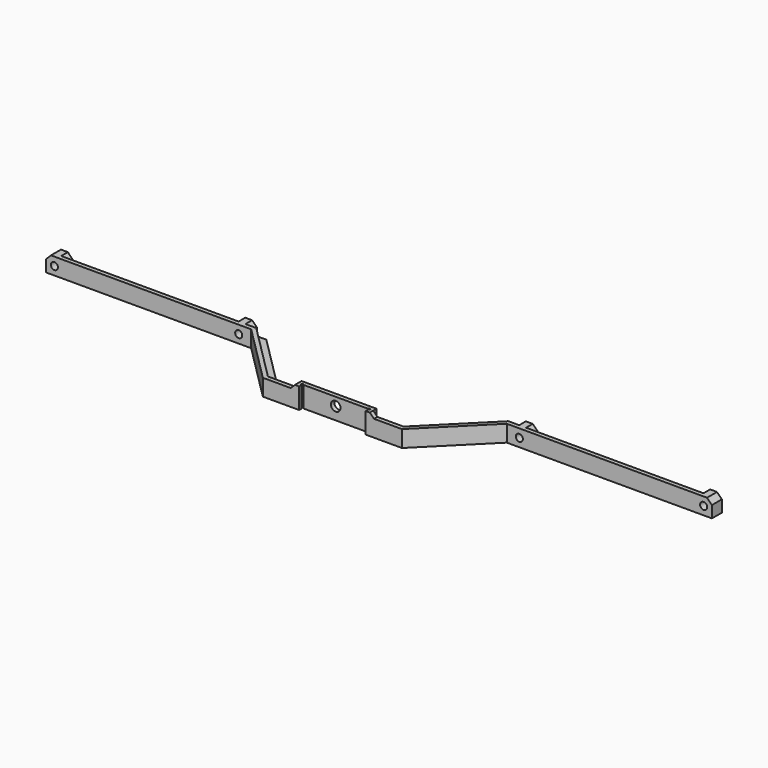
from build123d import *

# Parameters (mm, degrees)
F1_DEPTH  = 1.5875
F3_DEPTH  = 4.7625
F4_W      = 6.35
F4_H      = 6.35
F5_DEPTH  = 3.175
F6_SIZE   = 1.8598642
F7_W      = 28.575
F7_H      = 3.175
F8_DEPTH  = 1.5875
F9_W      = 25.4
F9_H      = 1.5875
F10_DEPTH = 7.9375
F11_R     = 1.35255
F11_R_2   = 1.8288
F12_DEPTH = 25.4
F13_SIZE  = 1.58749
F14_R     = 0.396875
F15_DEPTH = 7.9375


# Not quite as in the source:
# - a fillet or chamfer is up to 0.001 mm smaller than in the source, because OpenCascade refuses the exact size


with BuildPart() as f1:
    # F0 (on Top) → F1 (new body)
    with BuildSketch(Plane.XY):
        Polygon((-46.7826079092, 22.225), (-127, 22.225), (-127, 17.4625), (-48.7553, 17.4625), (-26.5303, -4.7625), (26.5303, -4.7625), (48.7553, 17.4625), (127, 17.4625), (127, 22.225), (46.7826079092, 22.225), (24.5576079092, 0), (-24.5576079092, 0), align=None)
    extrude(amount=F1_DEPTH)

    # F2 (on face) → F3 (join)
    with BuildSketch(Plane.XY.offset(1.5875)):
        Polygon((-127, 19.05), (-127, 17.4625), (-48.7553, 17.4625), (-26.5303, -4.7625), (26.5303, -4.7625), (48.7553, 17.4625), (127, 17.4625), (127, 19.05), (48.0977359697, 19.05), (25.8727359697, -3.175), (14.2875, -3.175), (14.2875, -1.5875), (-14.2875, -1.5875), (-14.2875, -3.175), (-25.8727359697, -3.175), (-48.0977359697, 19.05), align=None)
    extrude(amount=F3_DEPTH)

    # F4 (on face) → F5 (join, through all)
    with BuildSketch(Plane(origin=(0, 19.05, 0), x_dir=(-1, 0, 0), z_dir=(0, 1, 0))):
        with Locations((-53.5178, 3.175)):
            Rectangle(F4_W, F4_H)
        with Locations((-123.825, 3.175)):
            Rectangle(F4_W, F4_H)
        with Locations((123.825, 3.175)):
            Rectangle(F4_W, F4_H)
        with Locations((53.5178, 3.175)):
            Rectangle(F4_W, F4_H)
    extrude(amount=F5_DEPTH)

    # F6
    f6_edges = [f1.edges().sort_by_distance(p)[0] for p in [
        (-127, 19.84375, 6.35),
        (-120.65, 20.6375, 6.35),
        (-56.6928, 20.6375, 6.35),
        (-50.3428, 20.6375, 6.35),
        (50.3428, 20.6375, 6.35),
        (56.6928, 20.6375, 6.35),
        (120.65, 20.6375, 6.35),
        (127, 19.84375, 6.35),
    ]]
    chamfer(f6_edges, length=F6_SIZE)

    # F7 (on face) → F8 (join)
    with BuildSketch(Plane.XY.offset(6.35)):
        with Locations((0, -3.175)):
            Rectangle(F7_W, F7_H)
    extrude(amount=F8_DEPTH)

    # F9 (on face) → F10 (cut, through all)
    with BuildSketch(Plane.XY.offset(7.9375)):
        with Locations((0, -3.96875)):
            Rectangle(F9_W, F9_H)
    extrude(amount=-F10_DEPTH, mode=Mode.SUBTRACT)

    # F11 (on face) → F12 (cut, through all)
    with BuildSketch(Plane.XZ.offset(3.175)):
        with Locations((53.5178, 3.175)):
            Circle(F11_R)
        with Locations((123.825, 3.175)):
            Circle(F11_R)
        with Locations((-123.825, 3.175)):
            Circle(F11_R)
        with Locations((-53.5178, 3.175)):
            Circle(F11_R)
        with Locations((0, 4.7625)):
            Circle(F11_R_2)
    extrude(amount=-F12_DEPTH, mode=Mode.SUBTRACT)

    # F13 (size 1.5875 in the source; OpenCascade refuses exactly that, so slightly less here)
    f13_edges = [f1.edges().sort_by_distance(p)[0] for p in [
        (-14.2875, -3.96875, 6.35),
        (14.2875, -3.96875, 6.35),
    ]]
    chamfer(f13_edges, length=F13_SIZE)

    # F14 (on face) → F15 (cut, through all)
    with BuildSketch(Plane.XY.offset(7.9375)):
        with Locations((-12.7, -3.175)):
            Circle(F14_R)
        with Locations((12.7, -3.175)):
            Circle(F14_R)
    extrude(amount=-F15_DEPTH, mode=Mode.SUBTRACT)


solid = f1.part
